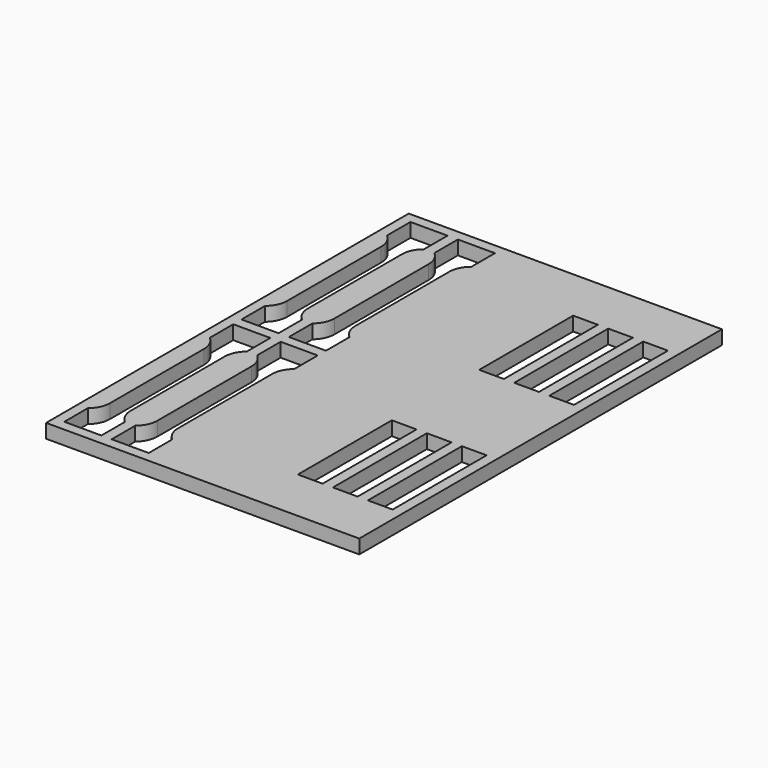
from build123d import *

# Parameters (mm, degrees)
F1_DEPTH = 110
F2_W     = 76
F2_H     = 8
F3_DEPTH = 152
F4_W     = 12
F4_H     = 57
F5_DEPTH = 152
F6_W     = 152
F6_H     = 220
F6_W_2   = 12
F6_H_2   = 57
F7_DEPTH = 145.2


# Not quite as in the source:
# - a feature names something its author has since deleted; it is built from what else it names


with BuildPart() as f1:
    # F0 (on Front) → F1 (new body, symmetric)
    with BuildSketch(Plane.XZ):
        with BuildLine():
            ThreePointArc((11.95, -69.2), (5.6567496474, -66.5932503526), (3.05, -60.3))
            Line((3.05, -60.3), (3.05, 60.3))
            ThreePointArc((3.05, 60.3), (5.6567496474, 66.5932503526), (11.95, 69.2))
            Line((11.95, 69.2), (76, 69.2))
            Line((76, 69.2), (76, 76))
            Line((76, 76), (-76, 76))
            Line((-76, 76), (-76, 69.2))
            Line((-76, 69.2), (-11.95, 69.2))
            ThreePointArc((-11.95, 69.2), (-5.6567496474, 66.5932503526), (-3.05, 60.3))
            Line((-3.05, 60.3), (-3.05, -60.3))
            ThreePointArc((-3.05, -60.3), (-5.6567496474, -66.5932503526), (-11.95, -69.2))
            Line((-11.95, -69.2), (-76, -69.2))
            Line((-76, -69.2), (-76, -76))
            Line((-76, -76), (76, -76))
            Line((76, -76), (76, -69.2))
            Line((76, -69.2), (11.95, -69.2))
        make_face()
    extrude(amount=F1_DEPTH, both=True)

    # F2 (on face) → F3 (join)
    with BuildSketch(Plane.XY.offset(76)):
        with Locations((-38, 0)):
            Rectangle(F2_W, F2_H)
    extrude(amount=-F3_DEPTH)

    # F4 (on face) → F5 (cut)
    with BuildSketch(Plane.XY.offset(76)):
        with BuildLine():
            ThreePointArc((-48.16667, 90.7352813742), (-45.2167956289, 86.9404157598), (-44.16667, 82.25))
            Line((-44.16667, 82.25), (-44.16667, 25.25))
            ThreePointArc((-44.16667, 25.25), (-45.2167956289, 20.5595842402), (-48.16667, 16.7647186258))
            Line((-48.16667, 16.7647186258), (-48.16667, 2.5))
            Line((-48.16667, 2.5), (-30.16667, 2.5))
            Line((-30.16667, 2.5), (-30.16667, 16.7647186258))
            ThreePointArc((-30.16667, 16.7647186258), (-33.1165443711, 20.5595842402), (-34.16667, 25.25))
            Line((-34.16667, 25.25), (-34.16667, 82.25))
            ThreePointArc((-34.16667, 82.25), (-33.1165443711, 86.9404157598), (-30.16667, 90.7352813742))
            Line((-30.16667, 90.7352813742), (-30.16667, 105))
            Line((-30.16667, 105), (-48.16667, 105))
            Line((-48.16667, 105), (-48.16667, 90.7352813742))
        make_face()
        with BuildLine():
            Line((-71.16667, 2.5), (-53.16667, 2.5))
            Line((-53.16667, 2.5), (-53.16667, 16.7647186258))
            ThreePointArc((-53.16667, 16.7647186258), (-56.1165443711, 20.5595842402), (-57.16667, 25.25))
            Line((-57.16667, 25.25), (-57.16667, 82.25))
            ThreePointArc((-57.16667, 82.25), (-56.1165443711, 86.9404157598), (-53.16667, 90.7352813742))
            Line((-53.16667, 90.7352813742), (-53.16667, 105))
            Line((-53.16667, 105), (-71.16667, 105))
            Line((-71.16667, 105), (-71.16667, 90.7352813742))
            ThreePointArc((-71.16667, 90.7352813742), (-68.2167956289, 86.9404157598), (-67.16667, 82.25))
            Line((-67.16667, 82.25), (-67.16667, 25.25))
            ThreePointArc((-67.16667, 25.25), (-68.2167956289, 20.5595842402), (-71.16667, 16.7647186258))
            Line((-71.16667, 16.7647186258), (-71.16667, 2.5))
        make_face()
        with Locations((31, 55)):
            Rectangle(F4_W, F4_H)
        with Locations((48, 55)):
            Rectangle(F4_W, F4_H)
        with Locations((65, 55)):
            Rectangle(F4_W, F4_H)
        with Locations((31, -55)):
            Rectangle(F4_W, F4_H)
        with Locations((48, -55)):
            Rectangle(F4_W, F4_H)
        with Locations((65, -55)):
            Rectangle(F4_W, F4_H)
        with BuildLine():
            Line((-71.16667, -105), (-53.16667, -105))
            Line((-53.16667, -105), (-53.16667, -90.7352813742))
            ThreePointArc((-53.16667, -90.7352813742), (-56.1165443711, -86.9404157598), (-57.16667, -82.25))
            Line((-57.16667, -82.25), (-57.16667, -25.25))
            ThreePointArc((-57.16667, -25.25), (-56.1165443711, -20.5595842402), (-53.16667, -16.7647186258))
            Line((-53.16667, -16.7647186258), (-53.16667, -2.5))
            Line((-53.16667, -2.5), (-71.16667, -2.5))
            Line((-71.16667, -2.5), (-71.16667, -16.7647186258))
            ThreePointArc((-71.16667, -16.7647186258), (-68.2167956289, -20.5595842402), (-67.16667, -25.25))
            Line((-67.16667, -25.25), (-67.16667, -82.25))
            ThreePointArc((-67.16667, -82.25), (-68.2167956289, -86.9404157598), (-71.16667, -90.7352813742))
            Line((-71.16667, -90.7352813742), (-71.16667, -105))
        make_face()
        with BuildLine():
            ThreePointArc((-48.16667, -16.7647186258), (-45.2167956289, -20.5595842402), (-44.16667, -25.25))
            Line((-44.16667, -25.25), (-44.16667, -82.25))
            ThreePointArc((-44.16667, -82.25), (-45.2167956289, -86.9404157598), (-48.16667, -90.7352813742))
            Line((-48.16667, -90.7352813742), (-48.16667, -105))
            Line((-48.16667, -105), (-30.16667, -105))
            Line((-30.16667, -105), (-30.16667, -90.7352813742))
            ThreePointArc((-30.16667, -90.7352813742), (-33.1165443711, -86.9404157598), (-34.16667, -82.25))
            Line((-34.16667, -82.25), (-34.16667, -25.25))
            ThreePointArc((-34.16667, -25.25), (-33.1165443711, -20.5595842402), (-30.16667, -16.7647186258))
            Line((-30.16667, -16.7647186258), (-30.16667, -2.5))
            Line((-30.16667, -2.5), (-48.16667, -2.5))
            Line((-48.16667, -2.5), (-48.16667, -16.7647186258))
        make_face()
    extrude(amount=-F5_DEPTH, mode=Mode.SUBTRACT)

    # F6 (on face) → F7 (cut)
    with BuildSketch(Plane(origin=(0, 0, -76), x_dir=(1, 0, 0), z_dir=(0, 0, -1))):
        Rectangle(F6_W, F6_H)
        with BuildLine():
            Line((-67.16667, -82.25), (-67.16667, -25.25))
            ThreePointArc((-67.16667, -25.25), (-68.2167956289, -20.5595842402), (-71.16667, -16.7647186258))
            Line((-71.16667, -16.7647186258), (-71.16667, -2.5))
            Line((-71.16667, -2.5), (-53.16667, -2.5))
            Line((-53.16667, -2.5), (-53.16667, -16.7647186258))
            ThreePointArc((-53.16667, -16.7647186258), (-56.1165443711, -20.5595842402), (-57.16667, -25.25))
            Line((-57.16667, -25.25), (-57.16667, -82.25))
            ThreePointArc((-57.16667, -82.25), (-56.1165443711, -86.9404157598), (-53.16667, -90.7352813742))
            Line((-53.16667, -90.7352813742), (-53.16667, -105))
            Line((-53.16667, -105), (-71.16667, -105))
            Line((-71.16667, -105), (-71.16667, -90.7352813742))
            ThreePointArc((-71.16667, -90.7352813742), (-68.2167956289, -86.9404157598), (-67.16667, -82.25))
        make_face(mode=Mode.SUBTRACT)
        with BuildLine():
            Line((-30.16667, -105), (-48.16667, -105))
            Line((-48.16667, -105), (-48.16667, -90.7352813742))
            ThreePointArc((-48.16667, -90.7352813742), (-45.2167956289, -86.9404157598), (-44.16667, -82.25))
            Line((-44.16667, -82.25), (-44.16667, -25.25))
            ThreePointArc((-44.16667, -25.25), (-45.2167956289, -20.5595842402), (-48.16667, -16.7647186258))
            Line((-48.16667, -16.7647186258), (-48.16667, -2.5))
            Line((-48.16667, -2.5), (-30.16667, -2.5))
            Line((-30.16667, -2.5), (-30.16667, -16.7647186258))
            ThreePointArc((-30.16667, -16.7647186258), (-33.1165443711, -20.5595842402), (-34.16667, -25.25))
            Line((-34.16667, -25.25), (-34.16667, -82.25))
            ThreePointArc((-34.16667, -82.25), (-33.1165443711, -86.9404157598), (-30.16667, -90.7352813742))
            Line((-30.16667, -90.7352813742), (-30.16667, -105))
        make_face(mode=Mode.SUBTRACT)
        with Locations((31, -55)):
            Rectangle(F6_W_2, F6_H_2, mode=Mode.SUBTRACT)
        with Locations((48, -55)):
            Rectangle(F6_W_2, F6_H_2, mode=Mode.SUBTRACT)
        with Locations((65, -55)):
            Rectangle(F6_W_2, F6_H_2, mode=Mode.SUBTRACT)
        with BuildLine():
            ThreePointArc((-67.16667, 82.25), (-68.2167956289, 86.9404157598), (-71.16667, 90.7352813742))
            Line((-71.16667, 90.7352813742), (-71.16667, 105))
            Line((-71.16667, 105), (-53.16667, 105))
            Line((-53.16667, 105), (-53.16667, 90.7352813742))
            ThreePointArc((-53.16667, 90.7352813742), (-56.1165443711, 86.9404157598), (-57.16667, 82.25))
            Line((-57.16667, 82.25), (-57.16667, 25.25))
            ThreePointArc((-57.16667, 25.25), (-56.1165443711, 20.5595842402), (-53.16667, 16.7647186258))
            Line((-53.16667, 16.7647186258), (-53.16667, 2.5))
            Line((-53.16667, 2.5), (-71.16667, 2.5))
            Line((-71.16667, 2.5), (-71.16667, 16.7647186258))
            ThreePointArc((-71.16667, 16.7647186258), (-68.2167956289, 20.5595842402), (-67.16667, 25.25))
            Line((-67.16667, 25.25), (-67.16667, 82.25))
        make_face(mode=Mode.SUBTRACT)
        with BuildLine():
            Line((-30.16667, 2.5), (-48.16667, 2.5))
            Line((-48.16667, 2.5), (-48.16667, 16.7647186258))
            ThreePointArc((-48.16667, 16.7647186258), (-45.2167956289, 20.5595842402), (-44.16667, 25.25))
            Line((-44.16667, 25.25), (-44.16667, 82.25))
            ThreePointArc((-44.16667, 82.25), (-45.2167956289, 86.9404157598), (-48.16667, 90.7352813742))
            Line((-48.16667, 90.7352813742), (-48.16667, 105))
            Line((-48.16667, 105), (-30.16667, 105))
            Line((-30.16667, 105), (-30.16667, 90.7352813742))
            ThreePointArc((-30.16667, 90.7352813742), (-33.1165443711, 86.9404157598), (-34.16667, 82.25))
            Line((-34.16667, 82.25), (-34.16667, 25.25))
            ThreePointArc((-34.16667, 25.25), (-33.1165443711, 20.5595842402), (-30.16667, 16.7647186258))
            Line((-30.16667, 16.7647186258), (-30.16667, 2.5))
        make_face(mode=Mode.SUBTRACT)
        with Locations((31, 55)):
            Rectangle(F6_W_2, F6_H_2, mode=Mode.SUBTRACT)
        with Locations((48, 55)):
            Rectangle(F6_W_2, F6_H_2, mode=Mode.SUBTRACT)
        with Locations((65, 55)):
            Rectangle(F6_W_2, F6_H_2, mode=Mode.SUBTRACT)
    extrude(amount=-F7_DEPTH, mode=Mode.SUBTRACT)


solid = f1.part
